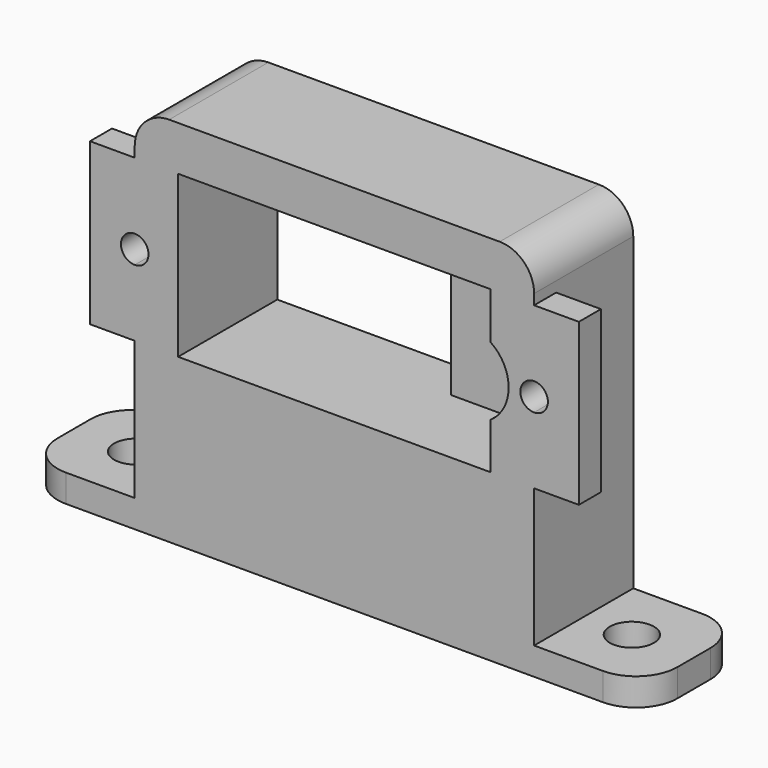
from build123d import *

# Parameters (mm, degrees)
F0_W      = 29
F0_H      = 9
F1_DEPTH  = 27
F0_W_2    = 8
F0_R      = 1.6
F2_DEPTH  = 2
F3_W      = 15
F3_H      = 11.7
F3_R      = 1.5
F4_DEPTH  = 10
F5_DEPTH  = 6
F6_DEPTH  = 7.5
F7_R      = 2.5
F8_R      = 3
F10_DEPTH = 2
F11_DEPTH = 3


# Not quite as in the source:
# - a feature names something its author has since deleted; it is built from what else it names


with BuildPart() as f1:
    # F0 (on Top) → F1 (new body)
    with BuildSketch(Plane.XY):
        with Locations((3.6698216572, -1.1730009172)):
            Rectangle(F0_W, F0_H)
    extrude(amount=F1_DEPTH)

    # F0 (on Top) → F2 (join)
    with BuildSketch(Plane.XY):
        with Locations((-14.8301783428, -1.1730009172)):
            Rectangle(F0_W_2, F0_H)
        with Locations((-14.3301783428, -1.1730009172)):
            Circle(F0_R, mode=Mode.SUBTRACT)
        with Locations((22.1698216572, -1.1730009172)):
            Rectangle(F0_W_2, F0_H)
        with Locations((21.6698216572, -1.1730009172)):
            Circle(F0_R, mode=Mode.SUBTRACT)
    extrude(amount=F2_DEPTH)

    # F3 (on face) → F4 (cut)
    with BuildSketch(Plane.XZ.offset(5.6730009172)):
        with Locations((-0.1801783428, 17.9)):
            Rectangle(F3_W, F3_H)
        with Locations((13.3198216572, 17.8843773901)):
            Circle(F3_R)
    extrude(amount=-F4_DEPTH, mode=Mode.SUBTRACT)

    # F3 (on face) → F5 (cut)
    with BuildSketch(Plane.XZ.offset(5.6730009172)):
        with BuildLine():
            Line((15.0198216572, 23.75), (7.3198216572, 23.75))
            Line((7.3198216572, 23.75), (7.3198216572, 12.05))
            Line((7.3198216572, 12.05), (15.0198216572, 12.05))
            Line((15.0198216572, 12.05), (15.0198216572, 15.4125359713))
            ThreePointArc((15.0198216572, 15.4125359713), (10.3198216572, 17.8843773901), (15.0198216572, 20.356218809))
            Line((15.0198216572, 20.356218809), (15.0198216572, 23.75))
        make_face()
    extrude(amount=-F5_DEPTH, mode=Mode.SUBTRACT)

    # F3 (on face) → F6 (cut)
    with BuildSketch(Plane.XZ.offset(5.6730009172)):
        with BuildLine():
            ThreePointArc((16.3198216572, 17.8843773901), (15.9750052667, 19.2808013945), (15.0198216572, 20.356218809))
            Line((15.0198216572, 20.356218809), (15.0198216572, 15.4125359713))
            ThreePointArc((15.0198216572, 15.4125359713), (15.9750052667, 16.4879533858), (16.3198216572, 17.8843773901))
        make_face()
        with BuildLine():
            Line((15.0198216572, 15.4125359713), (15.0198216572, 20.356218809))
            ThreePointArc((15.0198216572, 20.356218809), (10.3198216572, 17.8843773901), (15.0198216572, 15.4125359713))
        make_face()
        with Locations((13.3198216572, 17.8843773901)):
            Circle(F3_R, mode=Mode.SUBTRACT)
    extrude(amount=-F6_DEPTH, mode=Mode.SUBTRACT)

    # F7
    f7_edges = [f1.edges().sort_by_distance(p)[0] for p in [
        (-10.830178, -1.173001, 27),
        (18.169822, -1.173001, 27),
    ]]
    fillet(f7_edges, radius=F7_R)

    # F8
    f8_edges = [f1.edges().sort_by_distance(p)[0] for p in [
        (-18.830178, 3.326999, 1),
        (-18.830178, -5.673001, 1),
        (26.169822, -5.673001, 1),
        (26.169822, 3.326999, 1),
    ]]
    fillet(f8_edges, radius=F8_R)

    # F9 (on face) → F10 (join)
    with BuildSketch(Plane.XZ.offset(5.6730009172)):
        with BuildLine():
            Line((-14.0801783428, 12.05), (-10.8301783428, 12.05))
            Line((-10.8301783428, 12.05), (-10.8301783428, 16.9))
            ThreePointArc((-10.8301783428, 16.9), (-11.8301783428, 17.9), (-10.8301783428, 18.9))
            Line((-10.8301783428, 18.9), (-10.8301783428, 23.75))
            Line((-10.8301783428, 23.75), (-14.0801783428, 23.75))
            Line((-14.0801783428, 23.75), (-14.0801783428, 12.05))
        make_face()
        with BuildLine():
            Line((18.1698216572, 16.9), (18.1698216572, 12.05))
            Line((18.1698216572, 12.05), (21.4198216572, 12.05))
            Line((21.4198216572, 12.05), (21.4198216572, 23.75))
            Line((21.4198216572, 23.75), (18.1698216572, 23.75))
            Line((18.1698216572, 23.75), (18.1698216572, 18.9))
            ThreePointArc((18.1698216572, 18.9), (18.8769284384, 18.6071067812), (19.1698216572, 17.9))
            ThreePointArc((19.1698216572, 17.9), (18.8769284384, 17.1928932188), (18.1698216572, 16.9))
        make_face()
    extrude(amount=-F10_DEPTH)

    # F9 (on face) → F11 (cut)
    with BuildSketch(Plane.XZ.offset(5.6730009172)):
        with BuildLine():
            Line((-10.8301783428, 18.9), (-10.8301783428, 16.9))
            ThreePointArc((-10.8301783428, 16.9), (-10.1230715616, 17.1928932188), (-9.8301783428, 17.9))
            ThreePointArc((-9.8301783428, 17.9), (-10.1230715616, 18.6071067812), (-10.8301783428, 18.9))
        make_face()
        with BuildLine():
            ThreePointArc((18.1698216572, 18.9), (17.1698216572, 17.9), (18.1698216572, 16.9))
            Line((18.1698216572, 16.9), (18.1698216572, 18.9))
        make_face()
    extrude(amount=-F11_DEPTH, mode=Mode.SUBTRACT)


solid = f1.part
